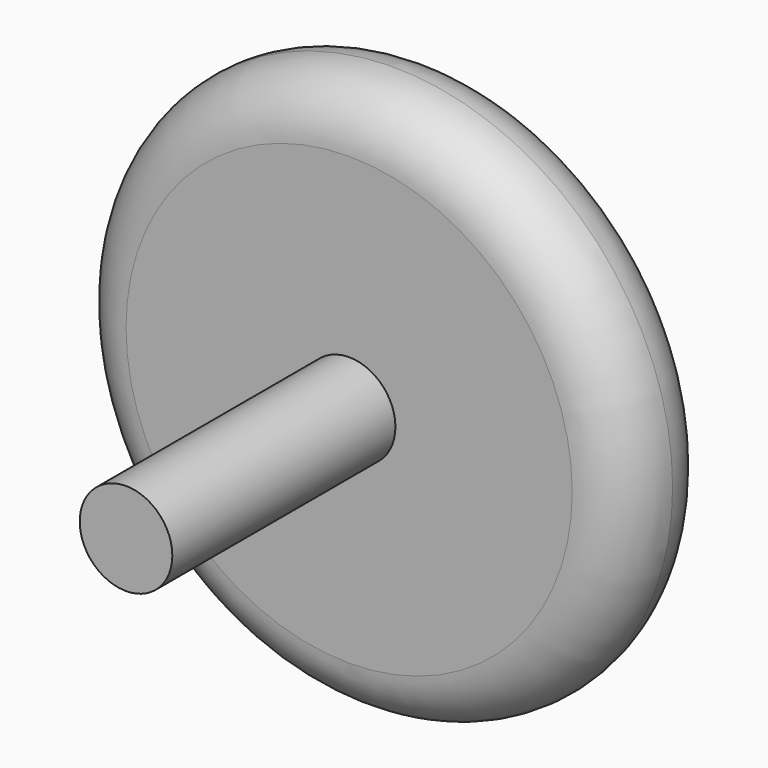
from build123d import *

# Parameters (mm, degrees)
F0_R     = 25.4
F1_DEPTH = 10.16
F2_R     = 5.08
F3_R     = 5.07999
F4_R     = 4.2168312207
F5_DEPTH = 25.4


# Not quite as in the source:
# - a fillet or chamfer is up to 0.001 mm smaller than in the source, because OpenCascade refuses the exact size


with BuildPart() as f1:
    # F0 (on Front) → F1 (new body)
    with BuildSketch(Plane.XZ):
        Circle(F0_R)
    extrude(amount=F1_DEPTH)

    # F2
    f2_edges = [f1.edges().sort_by_distance(p)[0] for p in [
        (-25.4, -10.16, 0),
    ]]
    fillet(f2_edges, radius=F2_R)

    # F3 (radius 5.08 in the source; OpenCascade refuses exactly that, so slightly less here)
    f3_edges = [f1.edges().sort_by_distance(p)[0] for p in [
        (-25.4, 0, 0),
    ]]
    fillet(f3_edges, radius=F3_R)

    # F4 (on face) → F5 (join)
    with BuildSketch(Plane.XZ.offset(10.16)):
        Circle(F4_R)
    extrude(amount=F5_DEPTH)


solid = f1.part
